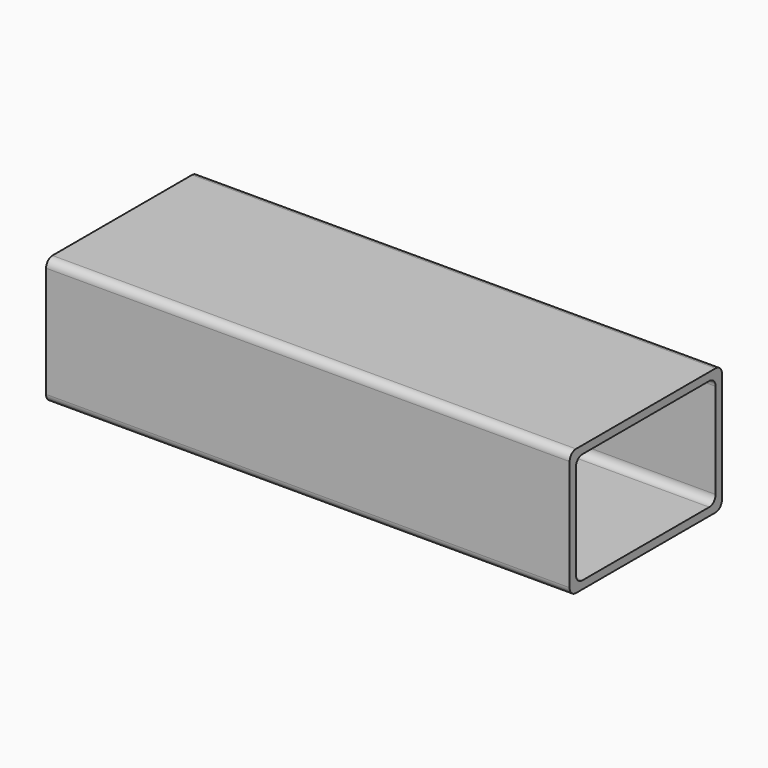
from build123d import *

# Parameters (mm, degrees)
F0_W     = 76.2
F0_H     = 50.8
F0_W_2   = 69.85
F0_H_2   = 44.45
F2_DEPTH = 209.55
F3_R     = 3.175


# Not quite as in the source:
# - a variable given as a bare number and used for a length is read in inches; the dataset says mm whatever the document's units were


with BuildPart() as f2:
    # F0 (on Right) → F2 (new body)
    with BuildSketch(Plane.YZ):
        Rectangle(F0_W, F0_H)
        Rectangle(F0_W_2, F0_H_2, mode=Mode.SUBTRACT)
    extrude(amount=F2_DEPTH)

    # F3
    f3_edges = [f2.edges().sort_by_distance(p)[0] for p in [
        (104.775, 38.1, 25.4),
        (104.775, 38.1, -25.4),
        (104.775, -38.1, -25.4),
        (104.775, -38.1, 25.4),
        (104.775, 34.925, -22.225),
        (104.775, 34.925, 22.225),
        (104.775, -34.925, 22.225),
        (104.775, -34.925, -22.225),
    ]]
    fillet(f3_edges, radius=F3_R)


solid = f2.part
